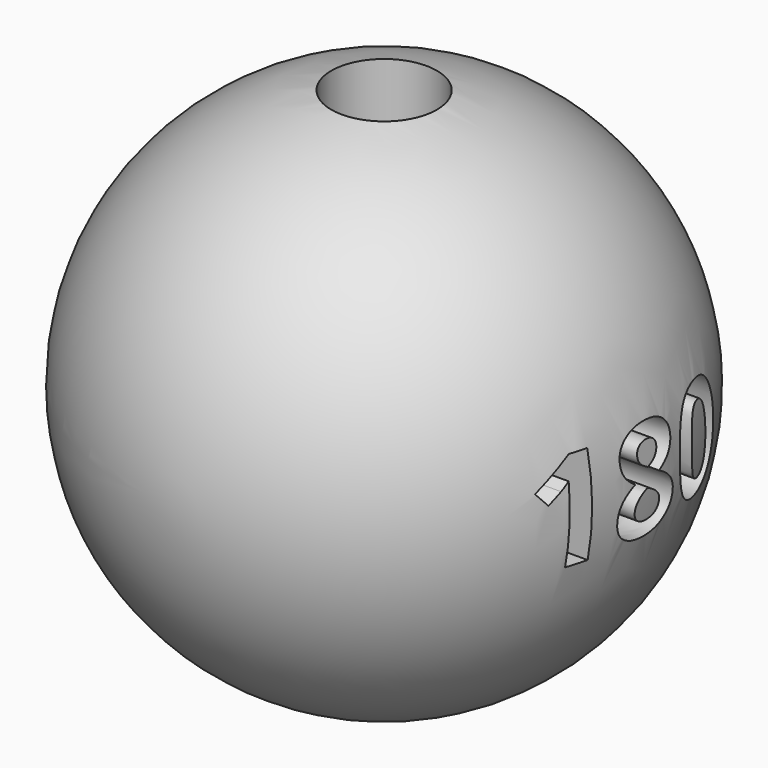
from build123d import *

# Parameters (mm, degrees)
F4_R          = 3.175
F5_DEPTH      = 25.4
F7_R          = 3.175
F5_FACE_R     = 3.175
F8_DEPTH      = 25.4
F12_TEXT_SIZE = 8.3017188849
F13_DEPTH     = 6.35


# Not quite as in the source:
# - a feature of the source that left no trace in its solid (it failed there, or was rolled back) is left out
# - Text() gives the source's letters only with a copy of the font that has no kerning and outlines rounded to 1/6400 em; it was checked with that copy


with BuildPart() as f2:
    # F1 (on Top) → F2 (revolve)
    with BuildSketch(Plane.XY):
        with BuildLine():
            Line((0, -15.875), (0, 15.875))
            ThreePointArc((0, 15.875), (-15.875, 0), (0, -15.875))
        make_face()
    revolve(axis=Axis((0, 0, 0), (0, -1, 0)))


with BuildPart() as f5:
    # F4 (on offset) → F5 (new body)
    with BuildSketch(Plane.XY.offset(6.35)):
        Circle(F4_R)
    extrude(amount=F5_DEPTH)


with BuildPart() as f8:
    # F7 (on offset) + F5_face (on face) → F8 (new body)
    with BuildSketch(Plane.XY.offset(-6.35)):
        Circle(F7_R)
    with BuildSketch(Plane.XY.offset(31.75)):
        Circle(F5_FACE_R)
    extrude(amount=-F8_DEPTH)


with BuildPart() as f2_1:
    add(f2.part)

    # F10: cut F5, F8
    add(f5.part, mode=Mode.SUBTRACT)
    add(f8.part, mode=Mode.SUBTRACT)

    # F12 (on offset) → F13 (cut)
    with BuildSketch(Plane.YZ.offset(16.51)):
        with Locations((-7.0954039693, -2.8941775672)):
            Text('180', F12_TEXT_SIZE, font='Open Sans', font_style=FontStyle.BOLD, text_align=(TextAlign.LEFT, TextAlign.BOTTOM))
    extrude(amount=-F13_DEPTH, mode=Mode.SUBTRACT)


solid = f2_1.part
